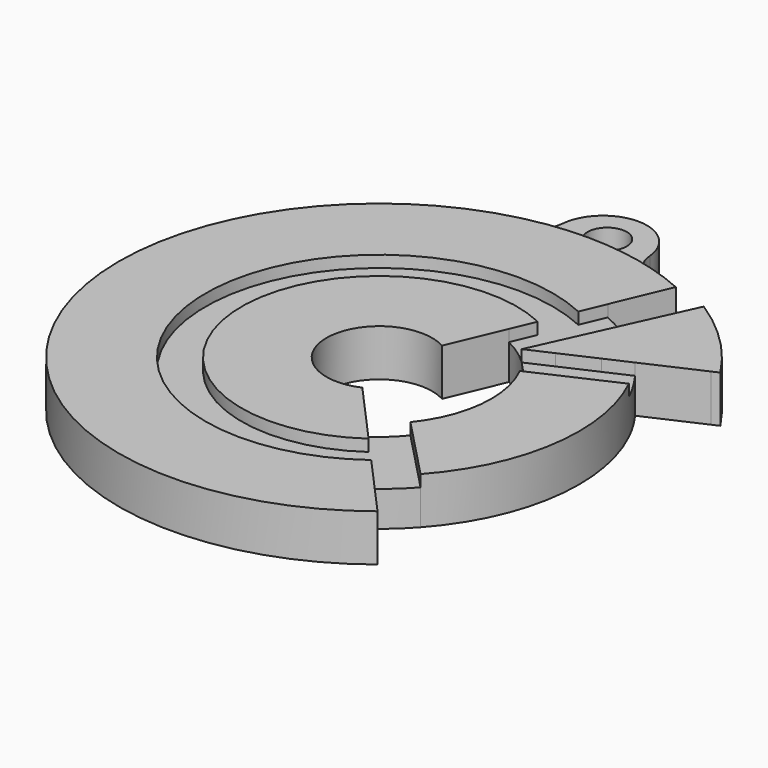
from build123d import *

# Parameters (mm, degrees)
F1_DEPTH    = 2.7
F2_DEPTH    = 0.9
F3_DEPTH    = 2.7
F4_DEPTH    = 0.9
F5_T1_DEPTH = 2.7
F6_DEPTH    = 0.9


# Not quite as in the source:
# - a fillet or chamfer that OpenCascade refuses, or shapes differently, is made with other operations: its cross-section is extruded or revolved along the edge and cut away or added
# - a feature of the source that left no trace in its solid (it failed there, or was rolled back) is left out


with BuildPart() as f1:
    # F0 (on Top) → F1 (new body)
    with BuildSketch(Plane.XY):
        with BuildLine():
            ThreePointArc((-2.9059050305, 19.7877668258), (-18.361479671, -7.928181651), (12.4102011034, -15.6839697964))
            Line((12.4102011034, -15.6839697964), (9.3065271924, -12.2254227754))
            ThreePointArc((9.3065271924, -12.2254227754), (-15.2699304913, -1.7034180964), (6.3836906961, 13.9757255095))
            Line((6.3836906961, 13.9757255095), (8.1864677167, 18.2477874364))
            ThreePointArc((8.1864677167, 18.2477874364), (5.5993809855, 19.2001805351), (2.9059050305, 19.7877668258))
            ThreePointArc((2.9059050305, 19.7877668258), (0, 18.1241204417), (-2.9059050305, 19.7877668258))
        make_face()
        with BuildLine():
            ThreePointArc((6.3836906961, 13.9757255095), (-15.2699304913, -1.7034180964), (9.3065271924, -12.2254227754))
            Line((9.3065271924, -12.2254227754), (7.9527661976, -10.7168731694))
            ThreePointArc((7.9527661976, -10.7168731694), (-13.2749249311, -1.3690247612), (5.5982117915, 12.114366903))
            Line((5.5982117915, 12.114366903), (6.3836906961, 13.9757255095))
        make_face()
        with BuildLine():
            ThreePointArc((5.5982117915, 12.114366903), (-13.2749249311, -1.3690247612), (7.9527661976, -10.7168731694))
            Line((7.9527661976, -10.7168731694), (6.0964799797, -8.6483397626))
            ThreePointArc((6.0964799797, -8.6483397626), (-10.5418803683, -0.9108276969), (4.5227579261, 9.5658512185))
            Line((4.5227579261, 9.5658512185), (5.5982117915, 12.114366903))
        make_face()
        with BuildLine():
            ThreePointArc((4.5227579261, 9.5658512185), (-10.5418803683, -0.9108276969), (6.0964799797, -8.6483397626))
            Line((6.0964799797, -8.6483397626), (4.7718042528, -7.1722010249))
            ThreePointArc((4.7718042528, -7.1722010249), (-8.5947223482, -0.5842355063), (3.7573171653, 7.7519772374))
            Line((3.7573171653, 7.7519772374), (4.5227579261, 9.5658512185))
        make_face()
        with BuildLine():
            ThreePointArc((3.7573171653, 7.7519772374), (-8.5947223482, -0.5842355063), (4.7718042528, -7.1722010249))
            Line((4.7718042528, -7.1722010249), (1.6593857385, -3.7039095455))
            ThreePointArc((1.6593857385, -3.7039095455), (-4.0546444127, 0.1799045205), (1.9809039535, 3.5423899386))
            Line((1.9809039535, 3.5423899386), (3.7573171653, 7.7519772374))
        make_face()
        with BuildLine():
            ThreePointArc((2.9059050305, 19.7877668258), (0, 20), (-2.9059050305, 19.7877668258))
            ThreePointArc((-2.9059050305, 19.7877668258), (0, 18.1241204417), (2.9059050305, 19.7877668258))
        make_face()
        with BuildLine():
            ThreePointArc((-3.157685128, 20.3174125427), (-3.043339046, 20.0471019762), (-2.9059050305, 19.7877668258))
            ThreePointArc((-2.9059050305, 19.7877668258), (0, 20), (2.9059050305, 19.7877668258))
            ThreePointArc((2.9059050305, 19.7877668258), (3.043339046, 20.0471019762), (3.157685128, 20.3174125427))
            ThreePointArc((3.157685128, 20.3174125427), (1.9207662081, 20.4714162913), (0.6767884164, 20.5501869879))
            ThreePointArc((0.6767884164, 20.5501869879), (0, 20.3893633928), (-0.6767884164, 20.5501869879))
            ThreePointArc((-0.6767884164, 20.5501869879), (-1.9207662081, 20.4714162913), (-3.157685128, 20.3174125427))
        make_face()
        with BuildLine():
            ThreePointArc((3.3697074825, 21.4938279241), (-0.5976844127, 24.8101062388), (-3.157685128, 20.3174125427))
            ThreePointArc((-3.157685128, 20.3174125427), (-1.9207662081, 20.4714162913), (-0.6767884164, 20.5501869879))
            ThreePointArc((-0.6767884164, 20.5501869879), (-0.7890530269, 23.1747685344), (1.5044645314, 21.8938279241))
            ThreePointArc((1.5044645314, 21.8938279241), (1.2809406102, 21.1047748972), (0.6767884164, 20.5501869879))
            ThreePointArc((0.6767884164, 20.5501869879), (1.9207662081, 20.4714162913), (3.157685128, 20.3174125427))
            ThreePointArc((3.157685128, 20.3174125427), (3.3162783146, 20.8961435115), (3.3697074825, 21.4938279241))
        make_face()
        with BuildLine():
            ThreePointArc((13.8344540426, 6.6843318112), (13.1730545976, 7.9084159596), (12.4036340143, 9.0676498421))
            Line((12.4036340143, 9.0676498421), (10.5172175152, 8.21498609))
            ThreePointArc((10.5172175152, 8.21498609), (11.318131065, 7.0709101194), (11.995098321, 5.8493997121))
            Line((11.995098321, 5.8493997121), (13.8344540426, 6.6843318112))
        make_face()
        with BuildLine():
            ThreePointArc((11.995098321, 5.8493997121), (11.318131065, 7.0709101194), (10.5172175152, 8.21498609))
            Line((10.5172175152, 8.21498609), (7.9045951482, 7.0340759404))
            ThreePointArc((7.9045951482, 7.0340759404), (8.7683299388, 5.9226040621), (9.4768887451, 4.706317935))
            Line((9.4768887451, 4.706317935), (11.995098321, 5.8493997121))
        make_face()
        with BuildLine():
            ThreePointArc((9.4768887451, 4.706317935), (8.7683299388, 5.9226040621), (7.9045951482, 7.0340759404))
            Line((7.9045951482, 7.0340759404), (6.0058132946, 6.1758230253))
            ThreePointArc((6.0058132946, 6.1758230253), (6.9398340598, 5.1038501734), (7.6848114732, 3.8928467719))
            Line((7.6848114732, 3.8928467719), (9.4768887451, 4.706317935))
        make_face()
        with BuildLine():
            Line((6.0058132946, 6.1758230253), (7.9045951482, 7.0340759404))
            ThreePointArc((7.9045951482, 7.0340759404), (7.4001814409, 7.5629467428), (6.8604632985, 8.0557365971))
            Line((6.8604632985, 8.0557365971), (6.0058132946, 6.1758230253))
        make_face()
        with BuildLine():
            ThreePointArc((6.8604632985, 8.0557365971), (5.7414756731, 8.8879866049), (4.5227579261, 9.5658512185))
            Line((4.5227579261, 9.5658512185), (3.7573171653, 7.7519772374))
            ThreePointArc((3.7573171653, 7.7519772374), (4.9447694202, 7.0540654058), (6.0058132946, 6.1758230253))
            Line((6.0058132946, 6.1758230253), (6.8604632985, 8.0557365971))
        make_face()
        with BuildLine():
            ThreePointArc((8.0404414582, 10.6512516579), (6.8584540657, 11.4481207432), (5.5982117915, 12.114366903))
            Line((5.5982117915, 12.114366903), (4.5227579261, 9.5658512185))
            ThreePointArc((4.5227579261, 9.5658512185), (5.7414756731, 8.8879866049), (6.8604632985, 8.0557365971))
            Line((6.8604632985, 8.0557365971), (8.0404414582, 10.6512516579))
        make_face()
        with BuildLine():
            ThreePointArc((8.8939895289, 12.5287413845), (7.6730254156, 13.3115397829), (6.3836906961, 13.9757255095))
            Line((6.3836906961, 13.9757255095), (5.5982117915, 12.114366903))
            ThreePointArc((5.5982117915, 12.114366903), (6.8584540657, 11.4481207432), (8.0404414582, 10.6512516579))
            Line((8.0404414582, 10.6512516579), (8.8939895289, 12.5287413845))
        make_face()
        with BuildLine():
            Line((7.9045951482, 7.0340759404), (10.5172175152, 8.21498609))
            ThreePointArc((10.5172175152, 8.21498609), (9.3584466725, 9.514059943), (8.0404414582, 10.6512516579))
            Line((8.0404414582, 10.6512516579), (6.8604632985, 8.0557365971))
            ThreePointArc((6.8604632985, 8.0557365971), (7.4001814409, 7.5629467428), (7.9045951482, 7.0340759404))
        make_face()
        with BuildLine():
            Line((10.5172175152, 8.21498609), (12.4036340143, 9.0676498421))
            ThreePointArc((12.4036340143, 9.0676498421), (10.7885115198, 10.9398550999), (8.8939895289, 12.5287413845))
            Line((8.8939895289, 12.5287413845), (8.0404414582, 10.6512516579))
            ThreePointArc((8.0404414582, 10.6512516579), (9.3584466725, 9.514059943), (10.5172175152, 8.21498609))
        make_face()
        with BuildLine():
            Line((12.4036340143, 9.0676498421), (16.6976556484, 11.008555575))
            ThreePointArc((16.6976556484, 11.008555575), (14.070563524, 14.2133473227), (10.8394114429, 16.807949297))
            Line((10.8394114429, 16.807949297), (8.8939895289, 12.5287413845))
            ThreePointArc((8.8939895289, 12.5287413845), (10.7885115198, 10.9398550999), (12.4036340143, 9.0676498421))
        make_face()
        with BuildLine():
            ThreePointArc((10.8394114429, 16.807949297), (14.070563524, 14.2133473227), (16.6976556484, 11.008555575))
            Line((16.6976556484, 11.008555575), (17.2154603994, 11.2426042817))
            ThreePointArc((17.2154603994, 11.2426042817), (14.4679762691, 14.6097874889), (11.0741551061, 17.3242984413))
            Line((11.0741551061, 17.3242984413), (10.8394114429, 16.807949297))
        make_face()
    extrude(amount=-F1_DEPTH)

    # F0 (on Top) → F2 (join)
    with BuildSketch(Plane.XY):
        with BuildLine():
            ThreePointArc((-2.9059050305, 19.7877668258), (-18.361479671, -7.928181651), (12.4102011034, -15.6839697964))
            Line((12.4102011034, -15.6839697964), (9.3065271924, -12.2254227754))
            ThreePointArc((9.3065271924, -12.2254227754), (-15.2699304913, -1.7034180964), (6.3836906961, 13.9757255095))
            Line((6.3836906961, 13.9757255095), (8.1864677167, 18.2477874364))
            ThreePointArc((8.1864677167, 18.2477874364), (5.5993809855, 19.2001805351), (2.9059050305, 19.7877668258))
            ThreePointArc((2.9059050305, 19.7877668258), (0, 18.1241204417), (-2.9059050305, 19.7877668258))
        make_face()
        with BuildLine():
            ThreePointArc((6.3836906961, 13.9757255095), (-15.2699304913, -1.7034180964), (9.3065271924, -12.2254227754))
            Line((9.3065271924, -12.2254227754), (7.9527661976, -10.7168731694))
            ThreePointArc((7.9527661976, -10.7168731694), (-13.2749249311, -1.3690247612), (5.5982117915, 12.114366903))
            Line((5.5982117915, 12.114366903), (6.3836906961, 13.9757255095))
        make_face()
        with BuildLine():
            ThreePointArc((4.5227579261, 9.5658512185), (-10.5418803683, -0.9108276969), (6.0964799797, -8.6483397626))
            Line((6.0964799797, -8.6483397626), (4.7718042528, -7.1722010249))
            ThreePointArc((4.7718042528, -7.1722010249), (-8.5947223482, -0.5842355063), (3.7573171653, 7.7519772374))
            Line((3.7573171653, 7.7519772374), (4.5227579261, 9.5658512185))
        make_face()
        with BuildLine():
            ThreePointArc((3.7573171653, 7.7519772374), (-8.5947223482, -0.5842355063), (4.7718042528, -7.1722010249))
            Line((4.7718042528, -7.1722010249), (1.6593857385, -3.7039095455))
            ThreePointArc((1.6593857385, -3.7039095455), (-4.0546444127, 0.1799045205), (1.9809039535, 3.5423899386))
            Line((1.9809039535, 3.5423899386), (3.7573171653, 7.7519772374))
        make_face()
        with BuildLine():
            ThreePointArc((2.9059050305, 19.7877668258), (0, 20), (-2.9059050305, 19.7877668258))
            ThreePointArc((-2.9059050305, 19.7877668258), (0, 18.1241204417), (2.9059050305, 19.7877668258))
        make_face()
    extrude(amount=F2_DEPTH)

    # F0 (on Top) → F3 (join)
    with BuildSketch(Plane.XY):
        with BuildLine():
            ThreePointArc((-2.9059050305, 19.7877668258), (-18.361479671, -7.928181651), (12.4102011034, -15.6839697964))
            Line((12.4102011034, -15.6839697964), (9.3065271924, -12.2254227754))
            ThreePointArc((9.3065271924, -12.2254227754), (-15.2699304913, -1.7034180964), (6.3836906961, 13.9757255095))
            Line((6.3836906961, 13.9757255095), (8.1864677167, 18.2477874364))
            ThreePointArc((8.1864677167, 18.2477874364), (5.5993809855, 19.2001805351), (2.9059050305, 19.7877668258))
            ThreePointArc((2.9059050305, 19.7877668258), (0, 18.1241204417), (-2.9059050305, 19.7877668258))
        make_face()
        with BuildLine():
            ThreePointArc((-3.157685128, 20.3174125427), (-3.043339046, 20.0471019762), (-2.9059050305, 19.7877668258))
            ThreePointArc((-2.9059050305, 19.7877668258), (0, 20), (2.9059050305, 19.7877668258))
            ThreePointArc((2.9059050305, 19.7877668258), (3.043339046, 20.0471019762), (3.157685128, 20.3174125427))
            ThreePointArc((3.157685128, 20.3174125427), (1.9207662081, 20.4714162913), (0.6767884164, 20.5501869879))
            ThreePointArc((0.6767884164, 20.5501869879), (0, 20.3893633928), (-0.6767884164, 20.5501869879))
            ThreePointArc((-0.6767884164, 20.5501869879), (-1.9207662081, 20.4714162913), (-3.157685128, 20.3174125427))
        make_face()
        with BuildLine():
            ThreePointArc((2.9059050305, 19.7877668258), (0, 20), (-2.9059050305, 19.7877668258))
            ThreePointArc((-2.9059050305, 19.7877668258), (0, 18.1241204417), (2.9059050305, 19.7877668258))
        make_face()
        with BuildLine():
            Line((7.9527661976, -10.7168731694), (9.3065271924, -12.2254227754))
            ThreePointArc((9.3065271924, -12.2254227754), (10.4014513861, -11.3085020883), (11.4065098197, -10.2938789654))
            Line((11.4065098197, -10.2938789654), (10.0042554899, -8.8324816906))
            ThreePointArc((10.0042554899, -8.8324816906), (9.0278120152, -9.8283503672), (7.9527661976, -10.7168731694))
        make_face()
        with BuildLine():
            ThreePointArc((6.3836906961, 13.9757255095), (-15.2699304913, -1.7034180964), (9.3065271924, -12.2254227754))
            Line((9.3065271924, -12.2254227754), (7.9527661976, -10.7168731694))
            ThreePointArc((7.9527661976, -10.7168731694), (-13.2749249311, -1.3690247612), (5.5982117915, 12.114366903))
            Line((5.5982117915, 12.114366903), (6.3836906961, 13.9757255095))
        make_face()
        with BuildLine():
            Line((12.4036340143, 9.0676498421), (16.6976556484, 11.008555575))
            ThreePointArc((16.6976556484, 11.008555575), (14.070563524, 14.2133473227), (10.8394114429, 16.807949297))
            Line((10.8394114429, 16.807949297), (8.8939895289, 12.5287413845))
            ThreePointArc((8.8939895289, 12.5287413845), (10.7885115198, 10.9398550999), (12.4036340143, 9.0676498421))
        make_face()
        with BuildLine():
            ThreePointArc((10.8394114429, 16.807949297), (14.070563524, 14.2133473227), (16.6976556484, 11.008555575))
            Line((16.6976556484, 11.008555575), (17.2154603994, 11.2426042817))
            ThreePointArc((17.2154603994, 11.2426042817), (14.4679762691, 14.6097874889), (11.0741551061, 17.3242984413))
            Line((11.0741551061, 17.3242984413), (10.8394114429, 16.807949297))
        make_face()
        with BuildLine():
            ThreePointArc((3.3697074825, 21.4938279241), (-0.5976844127, 24.8101062388), (-3.157685128, 20.3174125427))
            ThreePointArc((-3.157685128, 20.3174125427), (-1.9207662081, 20.4714162913), (-0.6767884164, 20.5501869879))
            ThreePointArc((-0.6767884164, 20.5501869879), (-0.7890530269, 23.1747685344), (1.5044645314, 21.8938279241))
            ThreePointArc((1.5044645314, 21.8938279241), (1.2809406102, 21.1047748972), (0.6767884164, 20.5501869879))
            ThreePointArc((0.6767884164, 20.5501869879), (1.9207662081, 20.4714162913), (3.157685128, 20.3174125427))
            ThreePointArc((3.157685128, 20.3174125427), (3.3162783146, 20.8961435115), (3.3697074825, 21.4938279241))
        make_face()
        with BuildLine():
            ThreePointArc((8.8939895289, 12.5287413845), (7.6730254156, 13.3115397829), (6.3836906961, 13.9757255095))
            Line((6.3836906961, 13.9757255095), (5.5982117915, 12.114366903))
            ThreePointArc((5.5982117915, 12.114366903), (6.8584540657, 11.4481207432), (8.0404414582, 10.6512516579))
            Line((8.0404414582, 10.6512516579), (8.8939895289, 12.5287413845))
        make_face()
        with BuildLine():
            Line((10.0042554899, -8.8324816906), (11.4065098197, -10.2938789654))
            ThreePointArc((11.4065098197, -10.2938789654), (14.3410149492, -5.5143177862), (15.3646480734, 0))
            ThreePointArc((15.3646480734, 0), (14.9772148291, 3.4286216448), (13.8344540426, 6.6843318112))
            Line((13.8344540426, 6.6843318112), (11.995098321, 5.8493997121))
            ThreePointArc((11.995098321, 5.8493997121), (13.0033922255, 3.0016081275), (13.3453310458, 0))
            ThreePointArc((13.3453310458, 0), (12.4821464921, -4.721639511), (10.0042554899, -8.8324816906))
        make_face()
        with BuildLine():
            Line((6.0964799797, -8.6483397626), (7.9527661976, -10.7168731694))
            ThreePointArc((7.9527661976, -10.7168731694), (9.0278120152, -9.8283503672), (10.0042554899, -8.8324816906))
            Line((10.0042554899, -8.8324816906), (8.0821585416, -6.8293163715))
            ThreePointArc((8.0821585416, -6.8293163715), (7.1474232492, -7.8022554232), (6.0964799797, -8.6483397626))
        make_face()
        with BuildLine():
            ThreePointArc((5.5982117915, 12.114366903), (-13.2749249311, -1.3690247612), (7.9527661976, -10.7168731694))
            Line((7.9527661976, -10.7168731694), (6.0964799797, -8.6483397626))
            ThreePointArc((6.0964799797, -8.6483397626), (-10.5418803683, -0.9108276969), (4.5227579261, 9.5658512185))
            Line((4.5227579261, 9.5658512185), (5.5982117915, 12.114366903))
        make_face()
        with BuildLine():
            Line((10.5172175152, 8.21498609), (12.4036340143, 9.0676498421))
            ThreePointArc((12.4036340143, 9.0676498421), (10.7885115198, 10.9398550999), (8.8939895289, 12.5287413845))
            Line((8.8939895289, 12.5287413845), (8.0404414582, 10.6512516579))
            ThreePointArc((8.0404414582, 10.6512516579), (9.3584466725, 9.514059943), (10.5172175152, 8.21498609))
        make_face()
        with BuildLine():
            ThreePointArc((13.8344540426, 6.6843318112), (13.1730545976, 7.9084159596), (12.4036340143, 9.0676498421))
            Line((12.4036340143, 9.0676498421), (10.5172175152, 8.21498609))
            ThreePointArc((10.5172175152, 8.21498609), (11.318131065, 7.0709101194), (11.995098321, 5.8493997121))
            Line((11.995098321, 5.8493997121), (13.8344540426, 6.6843318112))
        make_face()
        with BuildLine():
            ThreePointArc((8.0404414582, 10.6512516579), (6.8584540657, 11.4481207432), (5.5982117915, 12.114366903))
            Line((5.5982117915, 12.114366903), (4.5227579261, 9.5658512185))
            ThreePointArc((4.5227579261, 9.5658512185), (5.7414756731, 8.8879866049), (6.8604632985, 8.0557365971))
            Line((6.8604632985, 8.0557365971), (8.0404414582, 10.6512516579))
        make_face()
        with BuildLine():
            Line((8.0821585416, -6.8293163715), (10.0042554899, -8.8324816906))
            ThreePointArc((10.0042554899, -8.8324816906), (12.4821464921, -4.721639511), (13.3453310458, 0))
            ThreePointArc((13.3453310458, 0), (13.0033922255, 3.0016081275), (11.995098321, 5.8493997121))
            Line((11.995098321, 5.8493997121), (9.4768887451, 4.706317935))
            ThreePointArc((9.4768887451, 4.706317935), (10.3013902205, 2.4170660555), (10.5811553619, 0))
            ThreePointArc((10.5811553619, 0), (9.9367857977, -3.6360881181), (8.0821585416, -6.8293163715))
        make_face()
        with BuildLine():
            Line((4.7718042528, -7.1722010249), (6.0964799797, -8.6483397626))
            ThreePointArc((6.0964799797, -8.6483397626), (7.1474232492, -7.8022554232), (8.0821585416, -6.8293163715))
            Line((8.0821585416, -6.8293163715), (6.7113864418, -5.4007291543))
            ThreePointArc((6.7113864418, -5.4007291543), (5.8095133427, -6.3608284122), (4.7718042528, -7.1722010249))
        make_face()
        with BuildLine():
            ThreePointArc((4.5227579261, 9.5658512185), (-10.5418803683, -0.9108276969), (6.0964799797, -8.6483397626))
            Line((6.0964799797, -8.6483397626), (4.7718042528, -7.1722010249))
            ThreePointArc((4.7718042528, -7.1722010249), (-8.5947223482, -0.5842355063), (3.7573171653, 7.7519772374))
            Line((3.7573171653, 7.7519772374), (4.5227579261, 9.5658512185))
        make_face()
        with BuildLine():
            Line((7.9045951482, 7.0340759404), (10.5172175152, 8.21498609))
            ThreePointArc((10.5172175152, 8.21498609), (9.3584466725, 9.514059943), (8.0404414582, 10.6512516579))
            Line((8.0404414582, 10.6512516579), (6.8604632985, 8.0557365971))
            ThreePointArc((6.8604632985, 8.0557365971), (7.4001814409, 7.5629467428), (7.9045951482, 7.0340759404))
        make_face()
        with BuildLine():
            ThreePointArc((11.995098321, 5.8493997121), (11.318131065, 7.0709101194), (10.5172175152, 8.21498609))
            Line((10.5172175152, 8.21498609), (7.9045951482, 7.0340759404))
            ThreePointArc((7.9045951482, 7.0340759404), (8.7683299388, 5.9226040621), (9.4768887451, 4.706317935))
            Line((9.4768887451, 4.706317935), (11.995098321, 5.8493997121))
        make_face()
        with BuildLine():
            ThreePointArc((6.8604632985, 8.0557365971), (5.7414756731, 8.8879866049), (4.5227579261, 9.5658512185))
            Line((4.5227579261, 9.5658512185), (3.7573171653, 7.7519772374))
            ThreePointArc((3.7573171653, 7.7519772374), (4.9447694202, 7.0540654058), (6.0058132946, 6.1758230253))
            Line((6.0058132946, 6.1758230253), (6.8604632985, 8.0557365971))
        make_face()
        with BuildLine():
            Line((6.7113864418, -5.4007291543), (8.0821585416, -6.8293163715))
            ThreePointArc((8.0821585416, -6.8293163715), (9.9367857977, -3.6360881181), (10.5811553619, 0))
            ThreePointArc((10.5811553619, 0), (10.3013902205, 2.4170660555), (9.4768887451, 4.706317935))
            Line((9.4768887451, 4.706317935), (7.6848114732, 3.8928467719))
            ThreePointArc((7.6848114732, 3.8928467719), (8.3788968801, 2.00116727), (8.6145564813, 0))
            ThreePointArc((8.6145564813, 0), (8.1248446428, -2.8631246741), (6.7113864418, -5.4007291543))
        make_face()
        with BuildLine():
            ThreePointArc((3.7573171653, 7.7519772374), (-8.5947223482, -0.5842355063), (4.7718042528, -7.1722010249))
            Line((4.7718042528, -7.1722010249), (1.6593857385, -3.7039095455))
            ThreePointArc((1.6593857385, -3.7039095455), (-4.0546444127, 0.1799045205), (1.9809039535, 3.5423899386))
            Line((1.9809039535, 3.5423899386), (3.7573171653, 7.7519772374))
        make_face()
        with BuildLine():
            Line((6.0058132946, 6.1758230253), (7.9045951482, 7.0340759404))
            ThreePointArc((7.9045951482, 7.0340759404), (7.4001814409, 7.5629467428), (6.8604632985, 8.0557365971))
            Line((6.8604632985, 8.0557365971), (6.0058132946, 6.1758230253))
        make_face()
        with BuildLine():
            ThreePointArc((9.4768887451, 4.706317935), (8.7683299388, 5.9226040621), (7.9045951482, 7.0340759404))
            Line((7.9045951482, 7.0340759404), (6.0058132946, 6.1758230253))
            ThreePointArc((6.0058132946, 6.1758230253), (6.9398340598, 5.1038501734), (7.6848114732, 3.8928467719))
            Line((7.6848114732, 3.8928467719), (9.4768887451, 4.706317935))
        make_face()
    extrude(amount=-F3_DEPTH)

    # F0 (on Top) → F4 (join)
    with BuildSketch(Plane.XY):
        with BuildLine():
            Line((10.0042554899, -8.8324816906), (11.4065098197, -10.2938789654))
            ThreePointArc((11.4065098197, -10.2938789654), (14.3410149492, -5.5143177862), (15.3646480734, 0))
            ThreePointArc((15.3646480734, 0), (14.9772148291, 3.4286216448), (13.8344540426, 6.6843318112))
            Line((13.8344540426, 6.6843318112), (11.995098321, 5.8493997121))
            ThreePointArc((11.995098321, 5.8493997121), (13.0033922255, 3.0016081275), (13.3453310458, 0))
            ThreePointArc((13.3453310458, 0), (12.4821464921, -4.721639511), (10.0042554899, -8.8324816906))
        make_face()
        with BuildLine():
            Line((8.0821585416, -6.8293163715), (10.0042554899, -8.8324816906))
            ThreePointArc((10.0042554899, -8.8324816906), (12.4821464921, -4.721639511), (13.3453310458, 0))
            ThreePointArc((13.3453310458, 0), (13.0033922255, 3.0016081275), (11.995098321, 5.8493997121))
            Line((11.995098321, 5.8493997121), (9.4768887451, 4.706317935))
            ThreePointArc((9.4768887451, 4.706317935), (10.3013902205, 2.4170660555), (10.5811553619, 0))
            ThreePointArc((10.5811553619, 0), (9.9367857977, -3.6360881181), (8.0821585416, -6.8293163715))
        make_face()
        with BuildLine():
            Line((6.7113864418, -5.4007291543), (8.0821585416, -6.8293163715))
            ThreePointArc((8.0821585416, -6.8293163715), (9.9367857977, -3.6360881181), (10.5811553619, 0))
            ThreePointArc((10.5811553619, 0), (10.3013902205, 2.4170660555), (9.4768887451, 4.706317935))
            Line((9.4768887451, 4.706317935), (7.6848114732, 3.8928467719))
            ThreePointArc((7.6848114732, 3.8928467719), (8.3788968801, 2.00116727), (8.6145564813, 0))
            ThreePointArc((8.6145564813, 0), (8.1248446428, -2.8631246741), (6.7113864418, -5.4007291543))
        make_face()
        with BuildLine():
            ThreePointArc((10.8394114429, 16.807949297), (14.070563524, 14.2133473227), (16.6976556484, 11.008555575))
            Line((16.6976556484, 11.008555575), (17.2154603994, 11.2426042817))
            ThreePointArc((17.2154603994, 11.2426042817), (14.4679762691, 14.6097874889), (11.0741551061, 17.3242984413))
            Line((11.0741551061, 17.3242984413), (10.8394114429, 16.807949297))
        make_face()
        with BuildLine():
            Line((6.0058132946, 6.1758230253), (7.9045951482, 7.0340759404))
            ThreePointArc((7.9045951482, 7.0340759404), (7.4001814409, 7.5629467428), (6.8604632985, 8.0557365971))
            Line((6.8604632985, 8.0557365971), (6.0058132946, 6.1758230253))
        make_face()
        with BuildLine():
            Line((7.9045951482, 7.0340759404), (10.5172175152, 8.21498609))
            ThreePointArc((10.5172175152, 8.21498609), (9.3584466725, 9.514059943), (8.0404414582, 10.6512516579))
            Line((8.0404414582, 10.6512516579), (6.8604632985, 8.0557365971))
            ThreePointArc((6.8604632985, 8.0557365971), (7.4001814409, 7.5629467428), (7.9045951482, 7.0340759404))
        make_face()
        with BuildLine():
            Line((10.5172175152, 8.21498609), (12.4036340143, 9.0676498421))
            ThreePointArc((12.4036340143, 9.0676498421), (10.7885115198, 10.9398550999), (8.8939895289, 12.5287413845))
            Line((8.8939895289, 12.5287413845), (8.0404414582, 10.6512516579))
            ThreePointArc((8.0404414582, 10.6512516579), (9.3584466725, 9.514059943), (10.5172175152, 8.21498609))
        make_face()
        with BuildLine():
            Line((12.4036340143, 9.0676498421), (16.6976556484, 11.008555575))
            ThreePointArc((16.6976556484, 11.008555575), (14.070563524, 14.2133473227), (10.8394114429, 16.807949297))
            Line((10.8394114429, 16.807949297), (8.8939895289, 12.5287413845))
            ThreePointArc((8.8939895289, 12.5287413845), (10.7885115198, 10.9398550999), (12.4036340143, 9.0676498421))
        make_face()
    extrude(amount=F4_DEPTH)

    # F5: fillet of radius 3 on 2 edges, made by hand

    # F5_s2 → F5_t1 (join)
    with BuildSketch(Plane.XY.offset(-2.7)):
        with BuildLine():
            ThreePointArc((5.5129894146, 19.2251644392), (4.0340965589, 20.1897997022), (3.3539587166, 21.8192345075))
            ThreePointArc((3.3539587166, 21.8192345075), (3.2906213347, 20.768059539), (2.9059050305, 19.7877668258))
            ThreePointArc((2.9059050305, 19.7877668258), (4.2188358916, 19.5499724736), (5.5129894146, 19.2251644392))
        make_face()
        with BuildLine():
            ThreePointArc((-5.5129894146, 19.2251644392), (-4.0340965589, 20.1897997022), (-3.3539587166, 21.8192345075))
            ThreePointArc((-3.3539587166, 21.8192345075), (-3.2906213347, 20.768059539), (-2.9059050305, 19.7877668258))
            ThreePointArc((-2.9059050305, 19.7877668258), (-4.2188358916, 19.5499724736), (-5.5129894146, 19.2251644392))
        make_face()
    extrude(amount=F5_T1_DEPTH)


with BuildPart() as f6:
    # F6 (new): a face of the model
    f6_faces = [f1.part.faces().sort_by_distance(p)[0] for p in [
        (11.5302934708, -1.5094822973, 0.9),
    ]]
    extrude(f6_faces, amount=F6_DEPTH)


with BuildPart() as f6b:
    # F6#2 (new): a face of the model
    f6_2_faces = [f1.part.faces().sort_by_distance(p)[0] for p in [
        (11.5759648362, 11.7245978836, 0.9),
    ]]
    extrude(f6_2_faces, amount=F6_DEPTH)


solid = f1.part
